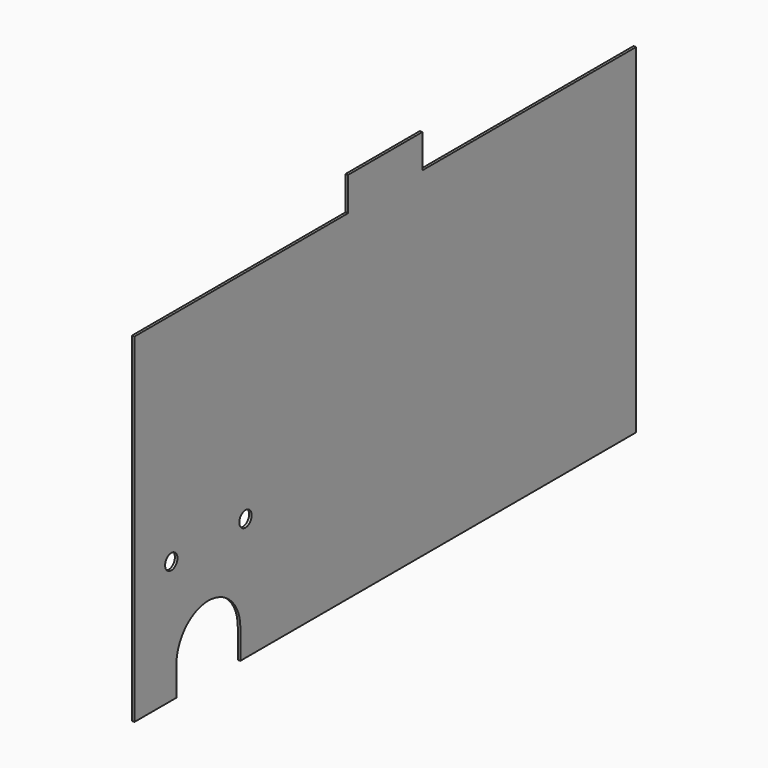
from build123d import *

# Parameters (mm, degrees)
F0_W     = 28.35
F0_H     = 108.95
F0_W_2   = 6
F0_H_2   = 28
F0_W_3   = 4
F0_H_3   = 32.75
F0_H_4   = 9.8
F0_H_5   = 24
F0_W_4   = 9.65
F0_H_6   = 76.2
F0_H_7   = 11.1
F0_R     = 3
F1_DEPTH = 1


# Not quite as in the source:
# - a feature names something its author has since deleted; it is built from what else it names


with BuildPart() as f1:
    # F0 (on Right) → F1 (new body)
    with BuildSketch(Plane.YZ):
        Polygon((178.337747033, -16.9212994559), (149.987747033, -16.9212994559), (130.337747033, -16.9212994559), (130.337747033, -39.6712994559), (251.987747033, -39.6712994559), (251.987747033, -16.9212994559), (182.337747033, -16.9212994559), align=None)
        with Locations((164.162747033, 37.5537005441)):
            Rectangle(F0_W, F0_H)
        Polygon((130.337747033, -16.9212994559), (149.987747033, -16.9212994559), (149.987747033, 92.0287005441), (148.337747033, 92.0287005441), (136.337747033, 92.0287005441), (136.337747033, 68.0287005441), (136.337747033, 56.9287005441), (136.337747033, 28.9287005441), (136.337747033, 19.1287005441), (136.337747033, -8.8712994559), (130.337747033, -8.8712994559), align=None)
        Polygon((130.337747033, -39.6712994559), (130.337747033, -16.9212994559), (110.687747033, -16.9212994559), (82.337747033, -16.9212994559), (82.337747033, -28.2962994559), (82.337747033, -39.6712994559), align=None)
        Polygon((110.687747033, -16.9212994559), (130.337747033, -16.9212994559), (130.337747033, -8.8712994559), (124.337747033, -8.8712994559), (124.337747033, 19.1287005441), (124.337747033, 21.9287005441), (124.337747033, 24.7287005441), (124.337747033, 27.5287005441), (124.337747033, 28.9287005441), (124.337747033, 56.9287005441), (130.337747033, 56.9287005441), (130.337747033, 68.0287005441), (124.337747033, 68.0287005441), (124.337747033, 92.0287005441), (130.337747033, 92.0287005441), (136.337747033, 92.0287005441), (148.337747033, 92.0287005441), (148.337747033, 102.1287005441), (148.337747033, 105.1287005441), (143.337747033, 105.1287005441), (130.337747033, 105.1287005441), (112.337747033, 105.1287005441), (112.337747033, 102.1287005441), (112.337747033, 92.0287005441), (110.687747033, 92.0287005441), align=None)
        Polygon((178.337747033, 92.0287005441), (178.337747033, -16.9212994559), (182.337747033, -16.9212994559), (182.337747033, 92.0287005441), (179.8798441887, 92.0287005441), align=None)
        Polygon((82.337747033, -16.9212994559), (110.687747033, -16.9212994559), (110.687747033, 92.0287005441), (82.337747033, 92.0287005441), (82.337747033, 15.8287005441), align=None)
        with Locations((133.337747033, 5.1287005441)):
            Rectangle(F0_W_2, F0_H_2)
        with Locations((127.337747033, 5.1287005441)):
            Rectangle(F0_W_2, F0_H_2)
        Polygon((182.337747033, 92.0287005441), (182.337747033, -16.9212994559), (251.987747033, -16.9212994559), (251.987747033, 92.0287005441), (226.687747033, 92.0287005441), (216.162747033, 92.0287005441), (214.687747033, 92.0287005441), align=None)
        Polygon((82.337747033, -28.2962994559), (82.337747033, -16.9212994559), (78.337747033, -16.9212994559), (68.687747033, -16.9212994559), (68.687747033, -28.2962994559), align=None)
        with Locations((80.337747033, -0.5462994559)):
            Rectangle(F0_W_3, F0_H_3)
        with Locations((133.337747033, 24.0287005441)):
            Rectangle(F0_W_2, F0_H_4)
        Polygon((124.337747033, 19.1287005441), (130.337747033, 19.1287005441), (130.337747033, 28.9287005441), (124.337747033, 28.9287005441), (124.337747033, 27.5287005441), (124.337747033, 24.7287005441), (124.337747033, 21.9287005441), align=None)
        Polygon((60.012747033, -39.6712994559), (82.337747033, -39.6712994559), (82.337747033, -28.2962994559), (68.687747033, -28.2962994559), (63.512747033, -28.2962994559), (60.012747033, -28.2962994559), align=None)
        with Locations((133.337747033, 80.0287005441)):
            Rectangle(F0_W_2, F0_H_5)
        with Locations((73.512747033, -0.5462994559)):
            Rectangle(F0_W_4, F0_H_3)
        with Locations((80.337747033, 53.9287005441)):
            Rectangle(F0_W_3, F0_H_6)
        with Locations((133.337747033, 42.9287005441)):
            Rectangle(F0_W_2, F0_H_2)
        with Locations((127.337747033, 42.9287005441)):
            Rectangle(F0_W_2, F0_H_2)
        with Locations((127.337747033, 80.0287005441)):
            Rectangle(F0_W_2, F0_H_5)
        with Locations((133.337747033, 62.4787005441)):
            Rectangle(F0_W_2, F0_H_7)
        with BuildLine():
            Line((68.687747033, -28.2962994559), (68.687747033, -16.9212994559))
            Line((68.687747033, -16.9212994559), (68.687747033, 15.8287005441))
            Line((68.687747033, 15.8287005441), (54.687747033, 15.8287005441))
            Line((54.687747033, 15.8287005441), (44.512747033, 15.8287005441))
            Line((44.512747033, 15.8287005441), (37.687747033, 15.8287005441))
            Line((37.687747033, 15.8287005441), (8.687747033, 15.8287005441))
            Line((8.687747033, 15.8287005441), (8.687747033, -28.2962994559))
            Line((8.687747033, -28.2962994559), (25.512747033, -28.2962994559))
            ThreePointArc((25.512747033, -28.2962994559), (31.0777181904, -14.8612706134), (44.512747033, -9.2962994559))
            ThreePointArc((44.512747033, -9.2962994559), (57.9477758755, -14.8612706134), (63.512747033, -28.2962994559))
            Line((63.512747033, -28.2962994559), (68.687747033, -28.2962994559))
        make_face()
        with Locations((26.512747033, 7.8287005441)):
            Circle(F0_R, mode=Mode.SUBTRACT)
        with BuildLine():
            ThreePointArc((59.512747033, 7.8287005441), (62.512747033, 10.8287005441), (65.512747033, 7.8287005441))
            ThreePointArc((65.512747033, 7.8287005441), (62.512747033, 4.8287005441), (59.512747033, 7.8287005441))
        make_face(mode=Mode.SUBTRACT)
        Polygon((68.687747033, 15.8287005441), (78.337747033, 15.8287005441), (78.337747033, 92.0287005441), (37.687747033, 92.0287005441), (8.687747033, 92.0287005441), (8.687747033, 32.6287005441), (33.187747033, 32.6287005441), (37.687747033, 32.6287005441), (37.687747033, 15.8287005441), (44.512747033, 15.8287005441), (54.687747033, 15.8287005441), align=None)
        with BuildLine():
            ThreePointArc((44.512747033, -12.7962994559), (55.4729021414, -17.3361443475), (60.012747033, -28.2962994559))
            Line((60.012747033, -28.2962994559), (63.512747033, -28.2962994559))
            ThreePointArc((63.512747033, -28.2962994559), (57.9477758755, -14.8612706134), (44.512747033, -9.2962994559))
            Line((44.512747033, -9.2962994559), (44.512747033, -12.7962994559))
        make_face()
        with BuildLine():
            ThreePointArc((29.012747033, -28.2962994559), (33.5525919246, -17.3361443475), (44.512747033, -12.7962994559))
            Line((44.512747033, -12.7962994559), (44.512747033, -9.2962994559))
            ThreePointArc((44.512747033, -9.2962994559), (31.0777181904, -14.8612706134), (25.512747033, -28.2962994559))
            Line((25.512747033, -28.2962994559), (28.8426652551, -28.2962994559))
            Line((28.8426652551, -28.2962994559), (29.012747033, -28.2962994559))
        make_face()
        Polygon((29.012747033, -39.6712994559), (29.012747033, -28.2962994559), (28.8426652551, -28.2962994559), (25.512747033, -28.2962994559), (8.687747033, -28.2962994559), (8.687747033, -39.6712994559), align=None)
        Polygon((33.187747033, 32.6287005441), (8.687747033, 32.6287005441), (8.687747033, 15.8287005441), (37.687747033, 15.8287005441), (37.687747033, 32.6287005441), align=None)
    extrude(amount=F1_DEPTH)


solid = f1.part
